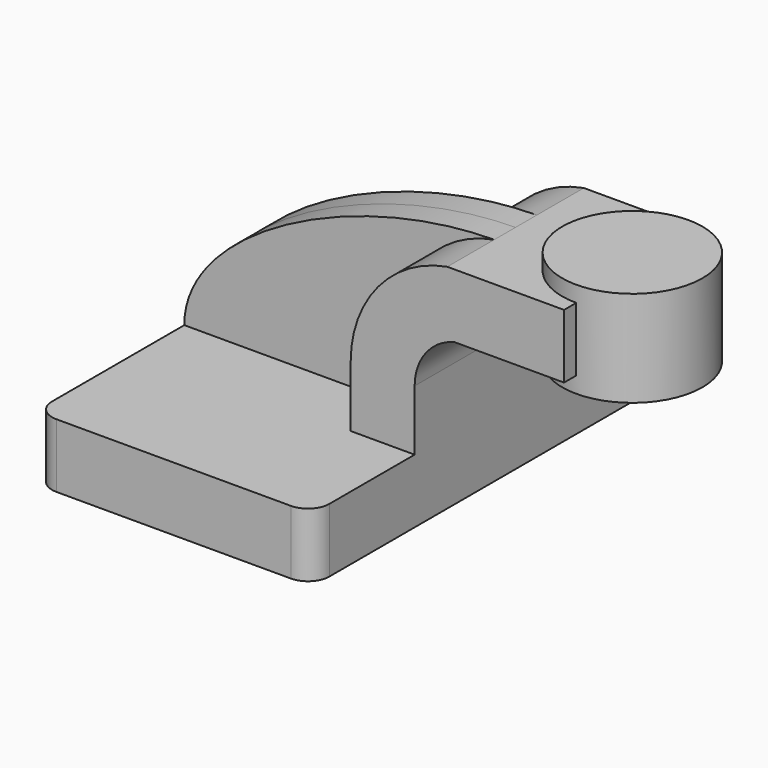
from build123d import *

# Parameters (mm, degrees)
F1_DEPTH = 63.5
F0_W     = 29.9330746515
F0_H     = 19.05
F2_DEPTH = 25.4
F3_DEPTH = 7.9375
F5_R     = 6.35


# Not quite as in the source:
# - the program builds the solid bodies; features that only make, move or delete a surface that nothing else refers to are left out


with BuildPart() as f1:
    # F0 (on Front) → F1 (new body, symmetric)
    with BuildSketch(Plane.XZ):
        Polygon((-41.275, 9.525), (-41.275, -9.525), (41.275, -9.525), (41.275, 9.525), (22.225, 9.525), align=None)
    extrude(amount=F1_DEPTH, both=True)

    # F0 (on Front) → F2 (join, symmetric)
    with BuildSketch(Plane.XZ):
        with BuildLine():
            Line((22.225, 9.525), (41.275, 9.525))
            Line((41.275, 9.525), (41.275, 27.5486753512))
            ThreePointArc((41.275, 27.5486753512), (44.5496824671, 37.2051562356), (53.0227320404, 42.8777746134))
            Line((53.0227320404, 42.8777746134), (55.8209344745, 42.8777746134))
            Line((55.8209344745, 42.8777746134), (55.8209344745, 61.9277746134))
            Line((55.8209344745, 61.9277746134), (50.9991334821, 61.9277746134))
            ThreePointArc((50.9991334821, 61.9277746134), (30.3677797958, 49.9644801757), (22.225, 27.5486753512))
            Line((22.225, 27.5486753512), (22.225, 9.525))
        make_face()
        with Locations((70.7874718002, 52.4027746134)):
            Rectangle(F0_W, F0_H)
    extrude(amount=F2_DEPTH, both=True)

    # F0 (on Front) → F3 (join, symmetric)
    with BuildSketch(Plane.XZ):
        with BuildLine():
            add(Edge.make_bspline(
                [(-41.275, 9.525), (-41.3442589343, 36.1172966659), (8.2413451746, 61.5874938667), (50.9991334821, 61.9277746134)],
                knots=[0, 0, 0, 0, 106.1158164321, 106.1158164321, 106.1158164321, 106.1158164321], degree=3))
            Line((-41.275, 9.525), (22.225, 9.525))
            Line((22.225, 9.525), (22.225, 27.5486753512))
            ThreePointArc((22.225, 27.5486753512), (30.3677797958, 49.9644801757), (50.9991334821, 61.9277746134))
        make_face()
    extrude(amount=F3_DEPTH, both=True)

    # F0 (on Front) → F4 (revolve)
    with BuildSketch(Plane.XZ):
        Polygon((85.754009126, 66.675), (85.754009126, 61.9277746134), (85.754009126, 42.8777746134), (85.754009126, 38.1), (106.6209344745, 38.1), (106.6209344745, 66.675), align=None)
    revolve(axis=Axis((85.754009126, 0, 52.3875), (0, 0, -1)))

    # F5
    f5_edges = [f1.edges().sort_by_distance(p)[0] for p in [
        (-41.275, -63.5, 0),
        (41.275, -63.5, 0),
        (-41.275, 63.5, 0),
        (41.275, 63.5, 0),
    ]]
    fillet(f5_edges, radius=F5_R)


solid = f1.part
